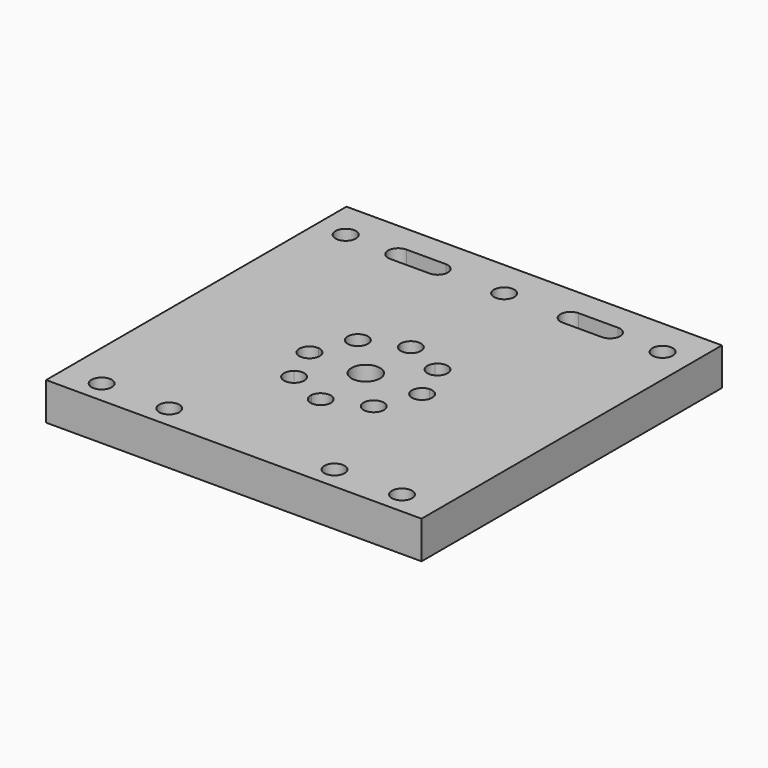
from build123d import *

# Parameters (mm, degrees)
F0_W     = 127
F0_H     = 127
F1_DEPTH = 12.7
F2_R     = 4.826
F3_DEPTH = 25.4
F4_R     = 3.429
F4_R_2   = 3.4577066483
F5_DEPTH = 25.4


# Not quite as in the source:
# - a feature names something its author has since deleted; it is built from what else it names


with BuildPart() as f1:
    # F0 (on Top) → F1 (new body)
    with BuildSketch(Plane.XY):
        Rectangle(F0_W, F0_H)
    extrude(amount=F1_DEPTH)

    # F2 (on face) → F3 (cut)
    with BuildSketch(Plane.XY.offset(12.7)):
        with BuildLine():
            ThreePointArc((-10.8373346815, 7.9672162229), (-15.8950533343, 8.195276323), (-15.6669932342, 3.1375576702))
            ThreePointArc((-15.6669932342, 3.1375576702), (-12.0167906073, 2.664949958), (-10.0413841816, 5.7706071703))
            ThreePointArc((-10.0413841816, 5.7706071703), (-10.2465070332, 6.9387925717), (-10.8373346815, 7.9672162229))
        make_face()
        with BuildLine():
            ThreePointArc((3.429, 11.3502229887), (-0.1544617901, 14.7757423005), (-3.4150843134, 11.0416129887))
            ThreePointArc((-3.4150843134, 11.0416129887), (0, 7.9212229887), (3.4150843134, 11.0416129887))
            ThreePointArc((3.4150843134, 11.0416129887), (3.4255193118, 11.1957611986), (3.429, 11.3502229887))
        make_face()
        with BuildLine():
            ThreePointArc((16.8993841816, 5.7706071703), (14.638569583, 8.9944843187), (10.8373346815, 7.9672162229))
            ThreePointArc((10.8373346815, 7.9672162229), (11.0457150289, 3.3459380176), (15.6669932342, 3.1375576702))
            ThreePointArc((15.6669932342, 3.1375576702), (16.576041394, 4.317013596), (16.8993841816, 5.7706071703))
        make_face()
        with BuildLine():
            ThreePointArc((22.479, -7.6997770113), (21.3629869552, -5.1683480976), (18.74139, -4.2846926978))
            ThreePointArc((18.74139, -4.2846926978), (15.621, -7.6997770113), (18.74139, -11.1148613247))
            ThreePointArc((18.74139, -11.1148613247), (21.3629869552, -10.231205925), (22.479, -7.6997770113))
        make_face()
        with BuildLine():
            ThreePointArc((15.6669932342, -18.5371116928), (11.0457150289, -18.7454920402), (10.8373346815, -23.3667702455))
            ThreePointArc((10.8373346815, -23.3667702455), (14.638569583, -24.3940383413), (16.8993841816, -21.1701611929))
            ThreePointArc((16.8993841816, -21.1701611929), (16.576041394, -19.7165676186), (15.6669932342, -18.5371116928))
        make_face()
        with BuildLine():
            ThreePointArc((3.4150843134, -26.4411670113), (0, -23.3207770113), (-3.4150843134, -26.4411670113))
            ThreePointArc((-3.4150843134, -26.4411670113), (-0.1544617901, -30.1752963231), (3.429, -26.7497770113))
            ThreePointArc((3.429, -26.7497770113), (3.4255193118, -26.5953152212), (3.4150843134, -26.4411670113))
        make_face()
        with BuildLine():
            ThreePointArc((-10.0413841816, -21.1701611929), (-12.0167906073, -18.0645039805), (-15.6669932342, -18.5371116928))
            ThreePointArc((-15.6669932342, -18.5371116928), (-15.8950533343, -23.5948303456), (-10.8373346815, -23.3667702455))
            ThreePointArc((-10.8373346815, -23.3667702455), (-10.2465070332, -22.3383465943), (-10.0413841816, -21.1701611929))
        make_face()
        with BuildLine():
            ThreePointArc((-15.621, -7.6997770113), (-16.5185710863, -5.3867900561), (-18.74139, -4.2846926978))
            ThreePointArc((-18.74139, -4.2846926978), (-22.479, -7.6997770113), (-18.74139, -11.1148613247))
            ThreePointArc((-18.74139, -11.1148613247), (-16.5185710863, -10.0127639665), (-15.621, -7.6997770113))
        make_face()
        with Locations((0, -7.6997770113)):
            Circle(F2_R)
    extrude(amount=-F3_DEPTH, mode=Mode.SUBTRACT)

    # F4 (on face) → F5 (cut)
    with BuildSketch(Plane.XY.offset(12.7)):
        with Locations((0, 50.8)):
            Circle(F4_R)
        with Locations((27.94, -55.88)):
            Circle(F4_R)
        with Locations((50.8, -55.88)):
            Circle(F4_R)
        with Locations((-50.8, -55.88)):
            Circle(F4_R)
        with Locations((-27.94, -55.88)):
            Circle(F4_R)
        with Locations((-53.594, 50.8)):
            Circle(F4_R_2)
        with Locations((53.594, 50.8)):
            Circle(F4_R_2)
        with BuildLine():
            Line((-22.479, 54.229), (-35.814, 54.229))
            ThreePointArc((-35.814, 54.229), (-39.243, 50.8), (-35.814, 47.371))
            Line((-35.814, 47.371), (-22.479, 47.371))
            ThreePointArc((-22.479, 47.371), (-19.05, 50.8), (-22.479, 54.229))
        make_face()
        with BuildLine():
            ThreePointArc((35.814, 47.371), (39.243, 50.8), (35.814, 54.229))
            Line((35.814, 54.229), (22.479, 54.229))
            ThreePointArc((22.479, 54.229), (19.05, 50.8), (22.479, 47.371))
            Line((22.479, 47.371), (35.814, 47.371))
        make_face()
    extrude(amount=-F5_DEPTH, mode=Mode.SUBTRACT)


solid = f1.part
